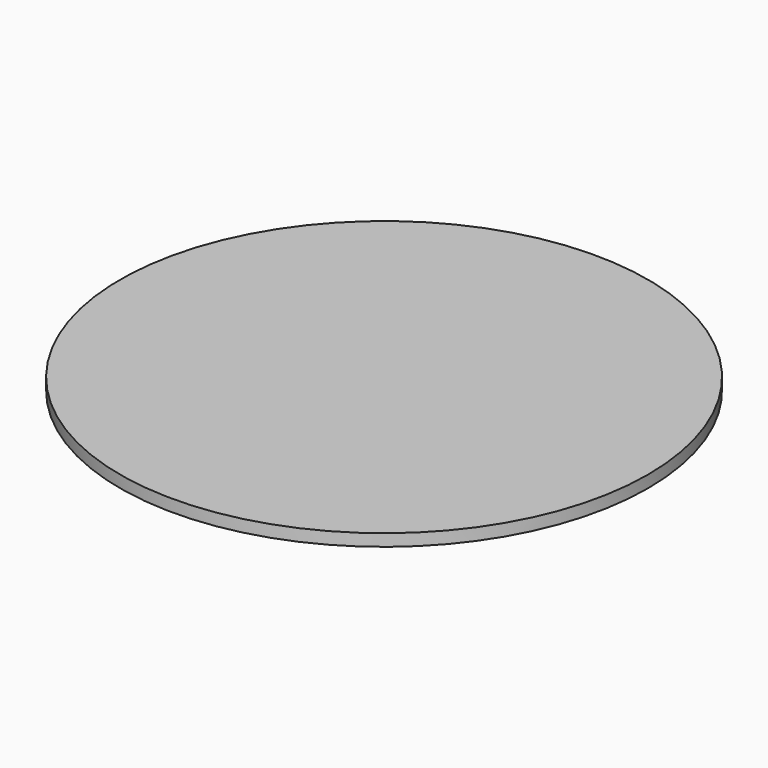
from build123d import *

# Parameters (mm, degrees)
F0_R     = 695.96
F0_R_2   = 675.64
F0_R_3   = 228.6
F0_R_4   = 199.2364019363
F0_R_5   = 152.4
F0_R_6   = 101.6
F1_DEPTH = 31.75


# Not quite as in the source:
# - the program builds the solid bodies; features that only make, move or delete a surface that nothing else refers to are left out


with BuildPart() as f1:
    # F0 (on Top) → F1 (new body)
    with BuildSketch(Plane.XY):
        Circle(F0_R)
        Circle(F0_R_2, mode=Mode.SUBTRACT)
        Circle(F0_R_2)
        Circle(F0_R_3, mode=Mode.SUBTRACT)
        Circle(F0_R_3)
        Circle(F0_R_4, mode=Mode.SUBTRACT)
        Circle(F0_R_4)
        Circle(F0_R_5, mode=Mode.SUBTRACT)
        Circle(F0_R_5)
        Circle(F0_R_6, mode=Mode.SUBTRACT)
        Circle(F0_R_6)
    extrude(amount=F1_DEPTH)


solid = f1.part
